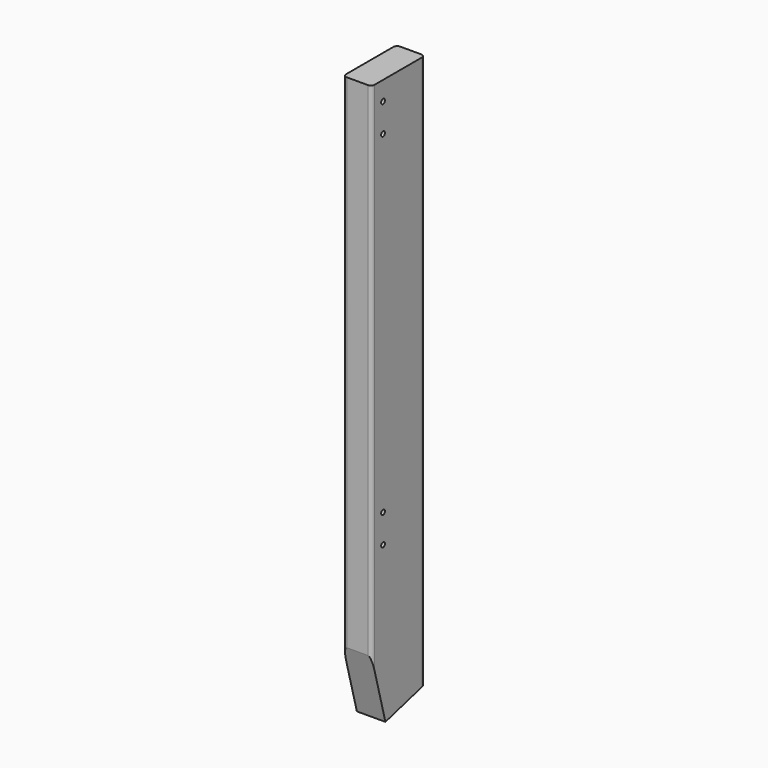
from build123d import *

# Parameters (mm, degrees)
F0_W     = 38.1
F0_H     = 88.9
F1_DEPTH = 381
F3_DEPTH = 38.101
F4_R     = 5.08
F6_D     = 6.35


# Not quite as in the source:
# - a feature names something its author has since deleted; it is built from what else it names


with BuildPart() as f1:
    # F0 (on Top) → F1 (new body, symmetric)
    with BuildSketch(Plane.XY):
        Rectangle(F0_W, F0_H)
    extrude(amount=F1_DEPTH, both=True)

    # F2 (on face) → F3 (cut, through all)
    with BuildSketch(Plane.YZ.offset(19.05)):
        Polygon((-21.4409868904, -374.8347535186), (-44.45, -381), (44.45, -381), (44.45, -357.1793167929), align=None)
        Polygon((-44.45, -288.9639475615), (-44.45, -381), (-21.4409868904, -374.8347535186), align=None)
    extrude(amount=-F3_DEPTH, mode=Mode.SUBTRACT)

    # F4
    f4_edges = [f1.edges().sort_by_distance(p)[0] for p in [
        (19.05, -44.45, 46.018026),
        (-19.05, -44.45, 46.018026),
        (19.05, 44.45, 11.910342),
        (-19.05, 44.45, 11.910342),
    ]]
    fillet(f4_edges, radius=F4_R)

    # F6 (through all)
    with Locations(Plane.YZ.offset(19.05)):
        with Locations((-25.4, 355.6), (-25.4, 317.5), (-25.4, -127), (-25.4, -165.1)):
            Hole(F6_D / 2)


solid = f1.part
